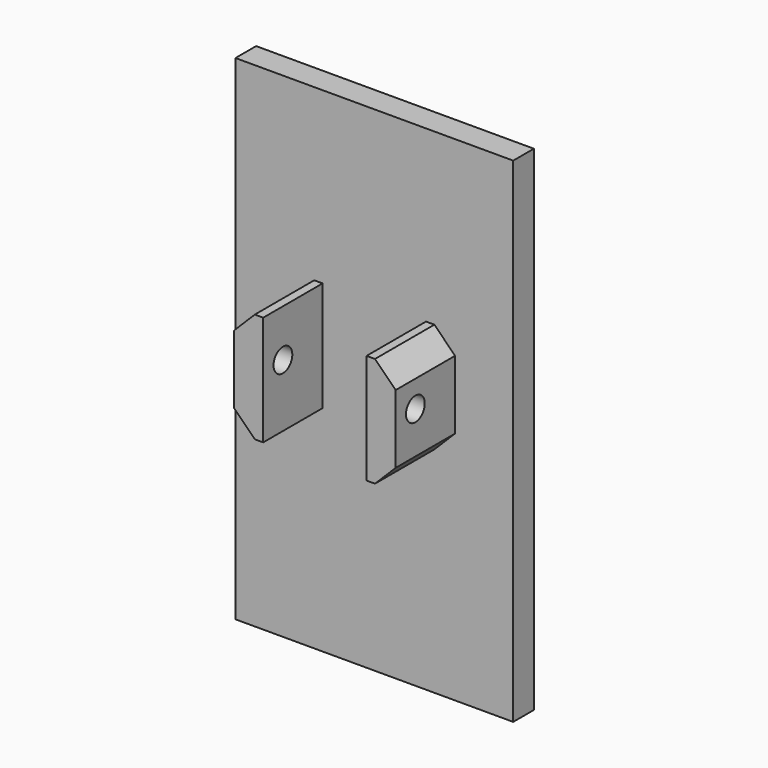
from build123d import *

# Parameters (mm, degrees)
F1_W      = 7.14375
F1_H      = 26.9875
F2_DEPTH  = 18.25625
F3_SIZE   = 5.08
F3_2_SIZE = 5.08
F4_R      = 2.8829
F5_DEPTH  = 50.8
F0_W      = 68.2625
F0_H      = 121.44375
F6_DEPTH  = 6.35


# Not quite as in the source:
# - a length typed as a fraction of an inch, garbled in the dataset ("3 / 203.2 mm" for 3/8 in), is restored


with BuildPart() as f2:
    # F1 (on Front) → F2 (new body)
    with BuildSketch(Plane.XZ):
        with Locations((16.2713638617, -0.3856395021)):
            Rectangle(F1_W, F1_H)
    extrude(amount=F2_DEPTH)

    # F3#2
    f3_2_edges = [f2.edges().sort_by_distance(p)[0] for p in [
        (19.843239, -9.128125, 13.10811),
        (19.843239, -9.128125, -13.87939),
    ]]
    chamfer(f3_2_edges, length=F3_2_SIZE)


with BuildPart() as f2b:
    # F1 (on Front) → F2, piece 2 (new body)
    with BuildSketch(Plane.XZ):
        with Locations((-16.2787499154, -0.3856395021)):
            Rectangle(F1_W, F1_H)
    extrude(amount=F2_DEPTH)

    # F3
    f3_edges = [f2b.edges().sort_by_distance(p)[0] for p in [
        (-19.850625, -9.128125, 13.10811),
        (-19.850625, -9.128125, -13.87939),
    ]]
    chamfer(f3_edges, length=F3_SIZE)


with BuildPart() as f5_tool:
    # F4 (on face) → F5 (new body)
    with BuildSketch(Plane(origin=(-19.8506249154, 0, 0), x_dir=(0, -1, 0), z_dir=(-1, 0, 0))):
        with Locations((12.19835, 1.4939604979)):
            Circle(F4_R)
    extrude(amount=-F5_DEPTH)


with BuildPart() as f2_1:
    add(f2.part)

    # F5: cut by f5_tool
    add(f5_tool.part, mode=Mode.SUBTRACT)


with BuildPart() as f2b_1:
    add(f2b.part)

    # F5: cut by f5_tool
    add(f5_tool.part, mode=Mode.SUBTRACT)


with BuildPart() as f6:
    # F0 (on Front) → F6 (new body)
    with BuildSketch(Plane.XZ):
        with Locations((0, -5.8215066612)):
            Rectangle(F0_W, F0_H)
    extrude(amount=-F6_DEPTH)


solid = Compound([f2_1.part, f2b_1.part, f6.part])
